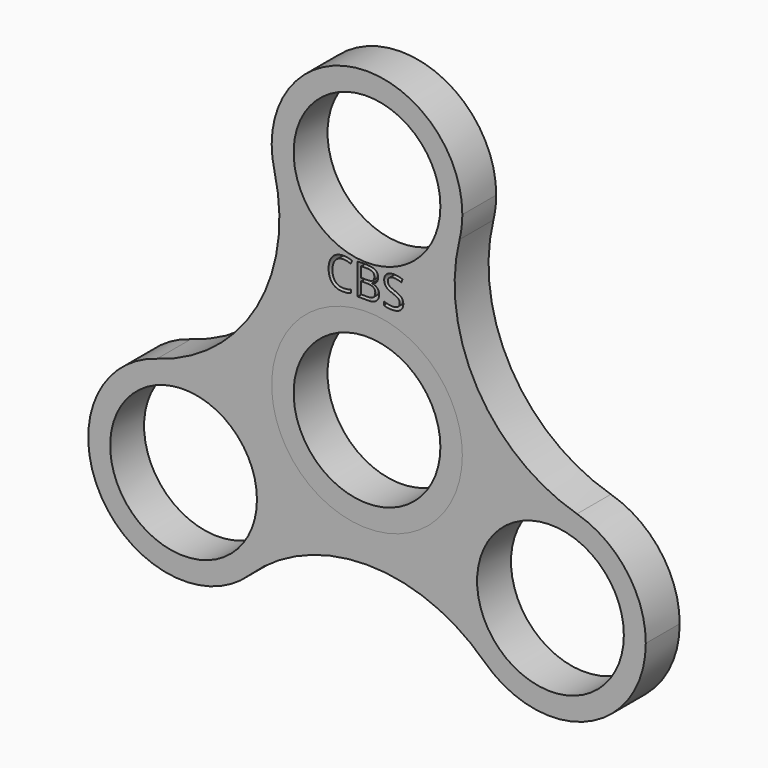
from build123d import *

# Parameters (mm, degrees)
F1_R         = 14.2875
F1_R_2       = 10.9982
F2_DEPTH     = 6.35
F0_R         = 14.2875
F0_R_2       = 10.9982
F3_TEXT_SIZE = 6.5128215485
F4_DEPTH     = 6.35


# Not quite as in the source:
# - Text() gives the source's letters only with a copy of the font that has no kerning and outlines rounded to 1/6400 em; it was checked with that copy


with BuildPart() as f2:
    # F1 (on Front) → F2 (new body)
    with BuildSketch(Plane.XZ):
        with BuildLine():
            ThreePointArc((31.4695122777, -2.1510686152), (16.5359438351, 9.5470316245), (13.8718760728, 28.3289313848))
            ThreePointArc((13.8718760728, 28.3289313848), (0, 17.4625), (-13.8718760728, 28.3289313848))
            ThreePointArc((-13.8718760728, 28.3289313848), (-16.5359438351, 9.5470316245), (-31.4695122777, -2.1510686152))
            ThreePointArc((-31.4695122777, -2.1510686152), (-18.912441482, -4.4535326513), (-13.2088065702, -15.875))
            ThreePointArc((-13.2088065702, -15.875), (-14.3517276668, -21.4743483284), (-17.5976362049, -26.1778627696))
            ThreePointArc((-17.5976362049, -26.1778627696), (0, -19.094063249), (17.5976362049, -26.1778627696))
            ThreePointArc((17.5976362049, -26.1778627696), (15.1229686136, -8.73125), (31.4695122777, -2.1510686152))
        make_face()
        Circle(F1_R, mode=Mode.SUBTRACT)
        with BuildLine():
            ThreePointArc((-13.8718760728, 28.3289313848), (0, 17.4625), (13.8718760728, 28.3289313848))
            ThreePointArc((13.8718760728, 28.3289313848), (14.1832134166, 30.0268884454), (14.2875, 31.75))
            ThreePointArc((14.2875, 31.75), (-1.7231115546, 45.9332134166), (-13.8718760728, 28.3289313848))
        make_face()
        with Locations((0, 31.75)):
            Circle(F1_R_2, mode=Mode.SUBTRACT)
        with BuildLine():
            ThreePointArc((41.7838065702, -15.875), (38.9177739189, -7.2911349119), (31.4695122777, -2.1510686152))
            ThreePointArc((31.4695122777, -2.1510686152), (15.1229686136, -8.73125), (17.5976362049, -26.1778627696))
            ThreePointArc((17.5976362049, -26.1778627696), (33.0956548986, -29.0195789034), (41.7838065702, -15.875))
        make_face()
        with Locations((27.4963065702, -15.875)):
            Circle(F1_R_2, mode=Mode.SUBTRACT)
        with BuildLine():
            ThreePointArc((-13.2088065702, -15.875), (-18.912441482, -4.4535326513), (-31.4695122777, -2.1510686152))
            ThreePointArc((-31.4695122777, -2.1510686152), (-39.8696445267, -23.01875), (-17.5976362049, -26.1778627696))
            ThreePointArc((-17.5976362049, -26.1778627696), (-14.3517276668, -21.4743483284), (-13.2088065702, -15.875))
        make_face()
        with Locations((-27.4963065702, -15.875)):
            Circle(F1_R_2, mode=Mode.SUBTRACT)
    extrude(amount=F2_DEPTH)

    # F3 (on face) → F4 (cut)
    with BuildSketch(Plane.XZ.offset(6.35)):
        with Locations((-6.154615432, 15.8261545002)):
            Text('CBS', F3_TEXT_SIZE, font='Open Sans', text_align=(TextAlign.LEFT, TextAlign.BOTTOM))
    extrude(amount=-F4_DEPTH, mode=Mode.SUBTRACT)


with BuildPart() as f2b:
    # F0 (on Front) → F2, piece 2 (new body)
    with BuildSketch(Plane.XZ):
        Circle(F0_R)
        Circle(F0_R_2, mode=Mode.SUBTRACT)
    extrude(amount=F2_DEPTH)


solid = Compound([f2.part, f2b.part])
